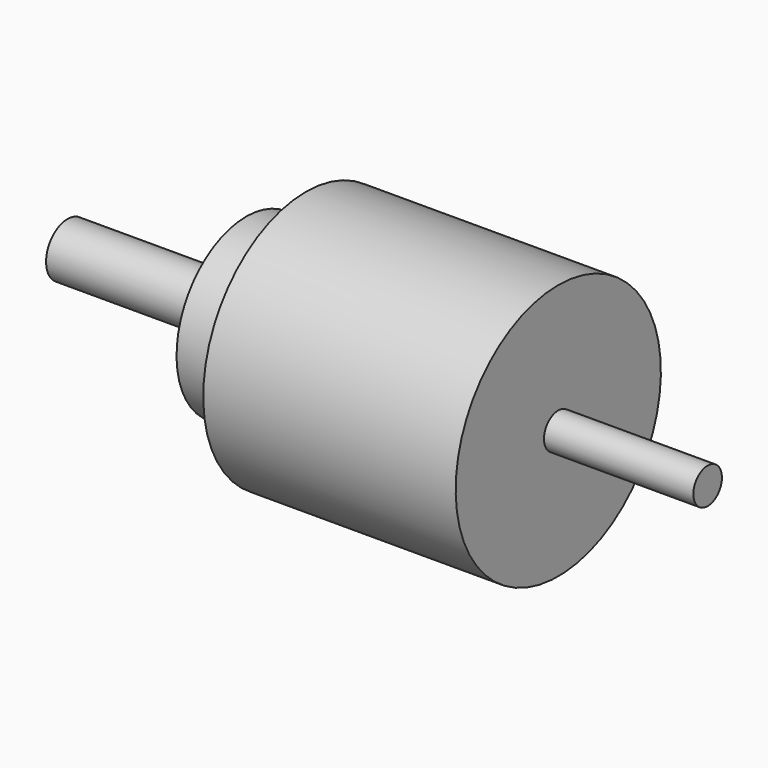
from build123d import *

# Parameters (mm, degrees)
F1_W = 16.71
F1_H = 2
F2_W = 50.41
F2_H = 2
F3_W = 20
F3_H = 3


with BuildPart() as f4:
    # F1 (on Front) → F4 (revolve)
    with BuildSketch(Plane.XZ):
        with Locations((8.355, 1)):
            Rectangle(F1_W, F1_H)
    revolve(axis=Axis((-19.1, 0, 0), (-1, 0, 0)))

    # F2 (on Front) → F5 (revolve)
    with BuildSketch(Plane.XZ):
        with Locations((-8.495, 1)):
            Rectangle(F2_W, F2_H)
    revolve(axis=Axis((-19.1, 0, 0), (-1, 0, 0)))


with BuildPart() as f4b:
    # F1 (on Front) → F4, piece 2 (revolve)
    with BuildSketch(Plane.XZ):
        Polygon((0, 14.35), (-28.2441887617, 14.35), (-30.9, 9.75), (-30.9, 2), (0, 2), align=None)
    revolve(axis=Axis((-19.1, 0, 0), (-1, 0, 0)))


with BuildPart() as f6:
    # F3 (on Front) → F6 (revolve)
    with BuildSketch(Plane.XZ):
        with Locations((-44.91, 1.5)):
            Rectangle(F3_W, F3_H)
        Polygon((-30.9, 9.75), (-34.91, 9.75), (-34.91, 3), (-34.91, 0), (-30.9, 0), align=None)
    revolve(axis=Axis((-19.1, 0, 0), (-1, 0, 0)))


solid = Compound([f4.part, f4b.part, f6.part])
